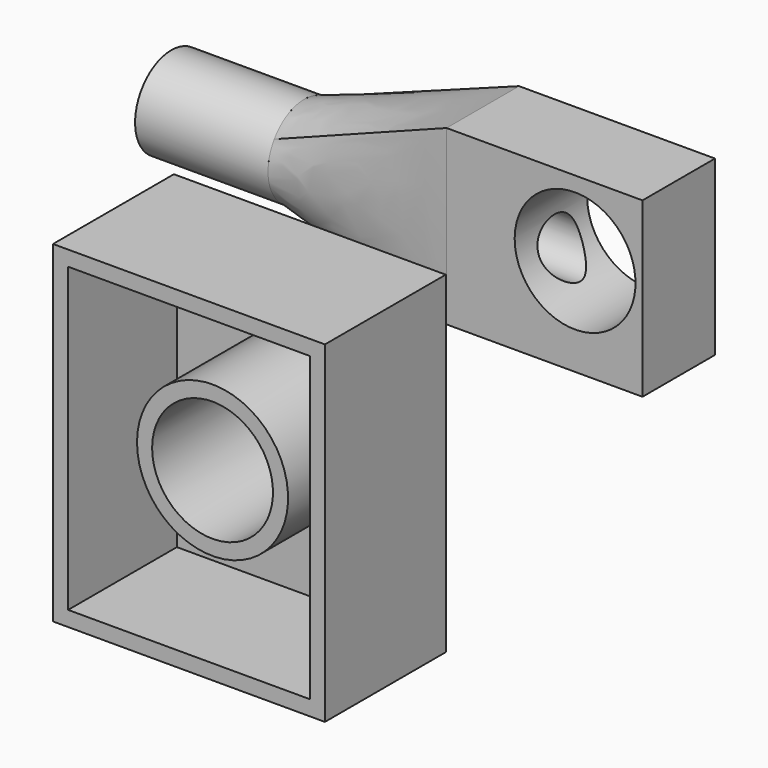
from build123d import *

# Parameters (mm, degrees)
F1_DEPTH  = 25
F4_W      = 32.4209956452
F4_H      = 28.6179427058
F5_DEPTH  = 15
F8_R      = 7.5
F9_DEPTH  = 22
F5_FACE_W = 15
F5_FACE_H = 28.6179427058
F12_R     = 5.1897115041
F13_DEPTH = 25
F14_R     = 10
F15_DEPTH = 200
F16_R     = 4.1944634135
F17_DEPTH = 80
F18_T     = -2.5


# Not quite as in the source:
# - the arcs of a loft's sections are written as splines that run evenly, so that the points pair up as in the source's solid
# - a feature names something its author has since deleted; it is built from what else it names
# - the program builds the solid bodies; features that only make, move or delete a surface that nothing else refers to are left out


with BuildPart() as f1:
    # F0 (on Front) → F1 (new body)
    with BuildSketch(Plane.XZ):
        Polygon((0, 55), (0, 0), (45, 0), (45, 55), (31.3274413347, 55), (12.6162180677, 55), align=None)
    extrude(amount=F1_DEPTH)

    # F12 (on face) → F13 (cut)
    with BuildSketch(Plane(origin=(44.024232716, 6.5541899568, 0), x_dir=(-0.1472539216, 0.9890987224, 0), z_dir=(0.9890987224, 0.1472539216, 0))):
        with Locations((18.0149693042, 30.8930817991)):
            Circle(F12_R)
    extrude(amount=-F13_DEPTH, mode=Mode.SUBTRACT)


with BuildPart() as f5:
    # F4 (on offset) → F5 (new body)
    with BuildSketch(Plane(origin=(0, 50, 0), x_dir=(-1, 0, 0), z_dir=(0, 1, 0))):
        with Locations((-21.3456586935, 28.7686688825)):
            Rectangle(F4_W, F4_H)
    extrude(amount=F5_DEPTH)

    # F5_face (on face) → F10 section 0
    with BuildSketch(Plane(origin=(5.1351608709, 57.5, 28.7686688825), x_dir=(0, -1, 0), z_dir=(-1, 0, 0))):
        Rectangle(F5_FACE_W, F5_FACE_H)
    # F9_face (on face) → F10 section 1
    with BuildSketch(Plane(origin=(-25, 58.2286454737, 26.6268867999), x_dir=(0, 1, 0), z_dir=(1, 0, 0))):
        with BuildLine():
            add(Edge.make_bspline(
                [(-4.2015845208, -6.2126232394), (-3.3883540404, -6.7626093671), (-2.4660875327, -7.1506811449), (-0.5424923825, -7.5445033349), (0.4580794074, -7.5500987948), (2.385958823, -7.177815061), (3.3125079103, -6.800082345), (4.9511694264, -5.7183695112), (5.6626371118, -5.0148150011), (6.2126232394, -4.2015845208)],
                knots=[0, 0, 0, 0, 0.25, 0.25, 0.5, 0.5, 0.75, 0.75, 1, 1, 1, 1], degree=3))
            add(Edge.make_bspline(
                [(6.2126232394, -4.2015845208), (6.7626093671, -3.3883540404), (7.1506811449, -2.4660875327), (7.5445033349, -0.5424923825), (7.5500987948, 0.4580794074), (7.177815061, 2.385958823), (6.800082345, 3.3125079103), (5.7183695112, 4.9511694264), (5.0148150011, 5.6626371118), (4.2015845208, 6.2126232394)],
                knots=[0, 0, 0, 0, 0.25, 0.25, 0.5, 0.5, 0.75, 0.75, 1, 1, 1, 1], degree=3))
            add(Edge.make_bspline(
                [(4.2015845208, 6.2126232394), (3.3883540404, 6.7626093671), (2.4660875327, 7.1506811449), (0.5424923825, 7.5445033349), (-0.4580794074, 7.5500987948), (-2.385958823, 7.177815061), (-3.3125079103, 6.800082345), (-4.9511694264, 5.7183695112), (-5.6626371118, 5.0148150011), (-6.2126232394, 4.2015845208)],
                knots=[0, 0, 0, 0, 0.25, 0.25, 0.5, 0.5, 0.75, 0.75, 1, 1, 1, 1], degree=3))
            add(Edge.make_bspline(
                [(-6.2126232394, 4.2015845208), (-6.7626093671, 3.3883540404), (-7.1506811449, 2.4660875327), (-7.5445033349, 0.5424923825), (-7.5500987948, -0.4580794074), (-7.177815061, -2.385958823), (-6.800082345, -3.3125079103), (-5.7183695112, -4.9511694264), (-5.0148150011, -5.6626371118), (-4.2015845208, -6.2126232394)],
                knots=[0, 0, 0, 0, 0.25, 0.25, 0.5, 0.5, 0.75, 0.75, 1, 1, 1, 1], degree=3))
        make_face()
    loft(ruled=True)


with BuildPart() as f9:
    # F8 (on offset) → F9 (new body)
    with BuildSketch(Plane.YZ.offset(-25)):
        with Locations((58.2286454737, 26.6268867999)):
            Circle(F8_R)
    extrude(amount=-F9_DEPTH)


with BuildPart() as f15_tool:
    # F14 (on face) → F15 (new body)
    with BuildSketch(Plane(origin=(0, 65, 0), x_dir=(-1, 0, 0), z_dir=(0, 1, 0))):
        with Locations((-26.4027472585, 30.6274686009)):
            Circle(F14_R)
    extrude(amount=-F15_DEPTH)


with BuildPart() as f1_1:
    add(f1.part)

    # F15: cut by f15_tool
    add(f15_tool.part, mode=Mode.SUBTRACT)

    # F18
    f18_openings = [f1_1.faces().sort_by_distance(p)[0] for p in [
        (0.710634, -25, 27.5),
    ]]
    offset(amount=F18_T, openings=f18_openings)


with BuildPart() as f5_1:
    add(f5.part)

    # F15: cut by f15_tool
    add(f15_tool.part, mode=Mode.SUBTRACT)


with BuildPart() as f17_tool:
    # F16 (on face) → F17 (new body)
    with BuildSketch(Plane(origin=(-47, 0, 0), x_dir=(0, -1, 0), z_dir=(-1, 0, 0))):
        with Locations((-58.2286454737, 26.6268867999)):
            Circle(F16_R)
    extrude(amount=-F17_DEPTH)


with BuildPart() as f5_2:
    add(f5_1.part)

    # F17: cut by f17_tool
    add(f17_tool.part, mode=Mode.SUBTRACT)


with BuildPart() as f9_1:
    add(f9.part)

    # F17: cut by f17_tool
    add(f17_tool.part, mode=Mode.SUBTRACT)


solid = Compound([f1_1.part, f5_2.part, f9_1.part])
